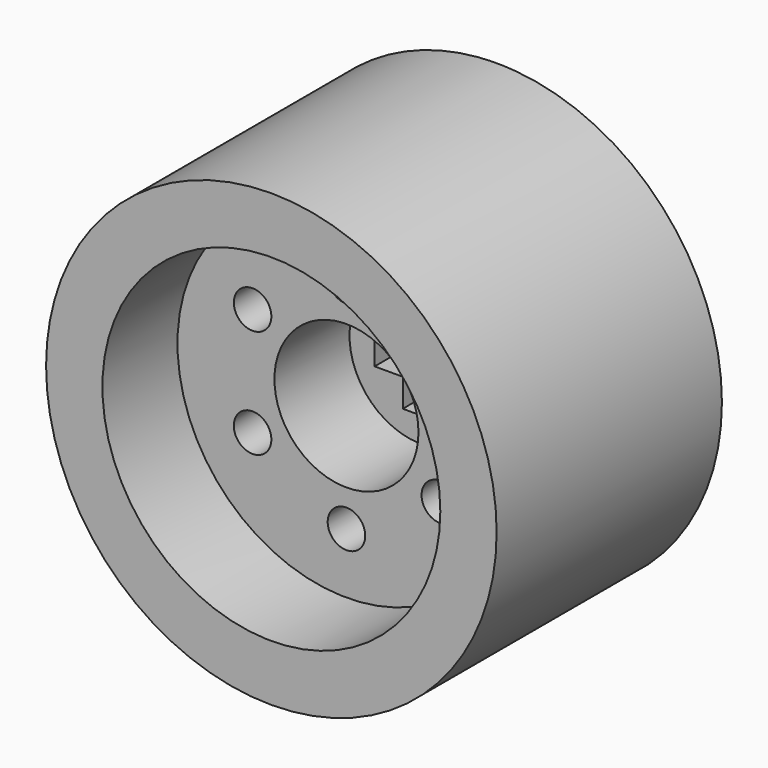
from build123d import *

# Parameters (mm, degrees)
F0_R     = 15.24
F0_R_2   = 12.7
F0_R_3   = 11.43
F1_DEPTH = 19.05
F0_R_4   = 1.27
F0_R_5   = 4.8718647292
F2_DEPTH = 12.7
F3_DEPTH = 6.35
F5_DEPTH = 7.62


# Not quite as in the source:
# - a feature of the source that left no trace in its solid (it failed there, or was rolled back) is left out
# - the program builds the solid bodies; features that only make, move or delete a surface that nothing else refers to are left out


with BuildPart() as f1:
    # F0 (on Front) → F1 (new body)
    with BuildSketch(Plane.XZ):
        Circle(F0_R)
        Circle(F0_R_2, mode=Mode.SUBTRACT)
        Circle(F0_R_2)
        Circle(F0_R_3, mode=Mode.SUBTRACT)
    extrude(amount=F1_DEPTH)

    # F0 (on Front) → F2 (join)
    with BuildSketch(Plane.XZ):
        Circle(F0_R_3)
        with Locations((-6.35, -3.6661742094)):
            Circle(F0_R_4, mode=Mode.SUBTRACT)
        with Locations((0, -7.3323484187)):
            Circle(F0_R_4, mode=Mode.SUBTRACT)
        with Locations((6.35, -3.6661742094)):
            Circle(F0_R_4, mode=Mode.SUBTRACT)
        with Locations((-6.35, 3.6661742094)):
            Circle(F0_R_4, mode=Mode.SUBTRACT)
        Circle(F0_R_5, mode=Mode.SUBTRACT)
        with Locations((6.35, 3.6661742094)):
            Circle(F0_R_4, mode=Mode.SUBTRACT)
        with Locations((0, 7.3323484187)):
            Circle(F0_R_4, mode=Mode.SUBTRACT)
    extrude(amount=F2_DEPTH)

    # F0 (on Front) → F3 (join)
    with BuildSketch(Plane.XZ):
        Circle(F0_R_5)
        Polygon((3.175, 1.27), (3.175, -1.27), (1.27, -1.27), (1.27, -3.175), (-1.27, -3.175), (-1.27, -1.27), (-3.175, -1.27), (-3.175, 1.27), (-1.27, 1.27), (-1.27, 3.175), (1.27, 3.175), (1.27, 1.27), align=None, mode=Mode.SUBTRACT)
        with Locations((6.35, 3.6661742094)):
            Circle(F0_R_4)
    extrude(amount=F3_DEPTH)

    # F0 (on Front) + F4 (on face) → F5 (join)
    with BuildSketch(Plane.XZ):
        with Locations((0, 7.3323484187)):
            Circle(F0_R_4)
        with Locations((6.35, -3.6661742094)):
            Circle(F0_R_4)
        with Locations((0, -7.3323484187)):
            Circle(F0_R_4)
        with Locations((-6.35, -3.6661742094)):
            Circle(F0_R_4)
        with Locations((-6.35, 3.6661742094)):
            Circle(F0_R_4)
    with BuildSketch(Plane(origin=(0, 0, 0), x_dir=(-1, 0, 0), z_dir=(0, 1, 0))):
        with BuildLine():
            ThreePointArc((-1.27, 7.3323484187), (0, 6.0623484187), (1.27, 7.3323484187))
            ThreePointArc((1.27, 7.3323484187), (0, 8.6023484187), (-1.27, 7.3323484187))
        make_face()
        with BuildLine():
            ThreePointArc((7.61993774, 3.678749442), (5.715, 4.7660264722), (5.7041406591, 2.5726634816))
            Line((5.7041406591, 2.5726634816), (7.61993774, 3.678749442))
        make_face()
        with BuildLine():
            Line((7.61993774, 3.678749442), (5.7041406591, 2.5726634816))
            ThreePointArc((5.7041406591, 2.5726634816), (6.9795469153, 2.5631915796), (7.62, 3.6661742094))
            ThreePointArc((7.62, 3.6661742094), (7.6199844349, 3.6724619027), (7.61993774, 3.678749442))
        make_face()
        with BuildLine():
            ThreePointArc((-1.27, 12.6363404513), (0, 12.7), (1.27, 12.6363404513))
            Line((1.27, 12.6363404513), (1.27, 15.1869911437))
            ThreePointArc((1.27, 15.1869911437), (0, 15.24), (-1.27, 15.1869911437))
            Line((-1.27, 15.1869911437), (-1.27, 12.6363404513))
        make_face()
        with BuildLine():
            Line((1.27, 15.1869911437), (1.27, 12.6363404513))
            ThreePointArc((1.27, 12.6363404513), (6.0659933949, 11.1576755703), (9.9146853041, 7.9365619333))
            Line((9.9146853041, 7.9365619333), (12.1355541331, 9.2187811496))
            ThreePointArc((12.1355541331, 9.2187811496), (7.3370363933, 13.3576007188), (1.27, 15.1869911437))
        make_face()
        with BuildLine():
            ThreePointArc((-11.4830868745, 5.4248240371), (-10.8829390696, 6.5461161927), (-10.1736532809, 7.6017615668))
            ThreePointArc((-10.1736532809, 7.6017615668), (-6.2510836052, 11.0550420063), (-1.27, 12.6363404513))
            Line((-1.27, 12.6363404513), (-1.27, 15.1869911437))
            ThreePointArc((-1.27, 15.1869911437), (-10.3175287739, -11.2163363002), (15.24, 0))
            ThreePointArc((15.24, 0), (14.7984009497, 3.6421050686), (13.4991956259, 7.0731405651))
            Line((13.4991956259, 7.0731405651), (11.2972745003, 5.8018608105))
            ThreePointArc((11.2972745003, 5.8018608105), (12.344338503, 2.9845111698), (12.7, 0))
            ThreePointArc((12.7, 0), (12.5183628333, -2.1402317572), (11.9786469332, -4.2192437297))
            ThreePointArc((11.9786469332, -4.2192437297), (11.4947402206, -5.4000877087), (10.8947701838, -6.5264065642))
            ThreePointArc((10.8947701838, -6.5264065642), (7.1599884636, -10.4892595163), (2.108859222, -12.5236860701))
            ThreePointArc((2.108859222, -12.5236860701), (0.843104089, -12.6719838816), (-0.431140778, -12.6926796867))
            ThreePointArc((-0.431140778, -12.6926796867), (-5.8966986399, -11.2480640623), (-10.1938394294, -7.5746707973))
            ThreePointArc((-10.1938394294, -7.5746707973), (-10.9002856113, -6.5171906211), (-11.4974295134, -5.3943595157))
            ThreePointArc((-11.4974295134, -5.3943595157), (-12.6999888406, 0.0168359612), (-11.4830868745, 5.4248240371))
        make_face()
        with BuildLine():
            Line((12.1355541331, 9.2187811496), (9.9146853041, 7.9365619333))
            ThreePointArc((9.9146853041, 7.9365619333), (10.6595519093, 6.9039085374), (11.2972745003, 5.8018608105))
            Line((11.2972745003, 5.8018608105), (13.4991956259, 7.0731405651))
            ThreePointArc((13.4991956259, 7.0731405651), (12.8621942988, 8.1744454135), (12.1355541331, 9.2187811496))
        make_face()
        with BuildLine():
            ThreePointArc((7.62, -3.6661742094), (6.5784622338, -2.4168924126), (5.1621968382, -3.2167038))
            Line((5.1621968382, -3.2167038), (7.3331543737, -4.4701067174))
            ThreePointArc((7.3331543737, -4.4701067174), (7.5461408894, -4.0929610094), (7.62, -3.6661742094))
        make_face()
        with BuildLine():
            Line((7.3331543737, -4.4701067174), (5.1621968382, -3.2167038))
            ThreePointArc((5.1621968382, -3.2167038), (5.715, -4.7660264722), (7.3331543737, -4.4701067174))
        make_face()
        with BuildLine():
            ThreePointArc((-5.08, -3.6661742094), (-5.4364655228, -2.7839300487), (-6.305755526, -2.3969451416))
            Line((-6.305755526, -2.3969451416), (-7.4713068529, -3.0698765139))
            ThreePointArc((-7.4713068529, -3.0698765139), (-6.6572786169, -4.8984403541), (-5.08, -3.6661742094))
        make_face()
        with BuildLine():
            Line((-7.4713068529, -3.0698765139), (-6.305755526, -2.3969451416))
            ThreePointArc((-6.305755526, -2.3969451416), (-6.985, -2.5663219465), (-7.4713068529, -3.0698765139))
        make_face()
    extrude(amount=F5_DEPTH, dir=(0, -1, 0))


solid = f1.part
